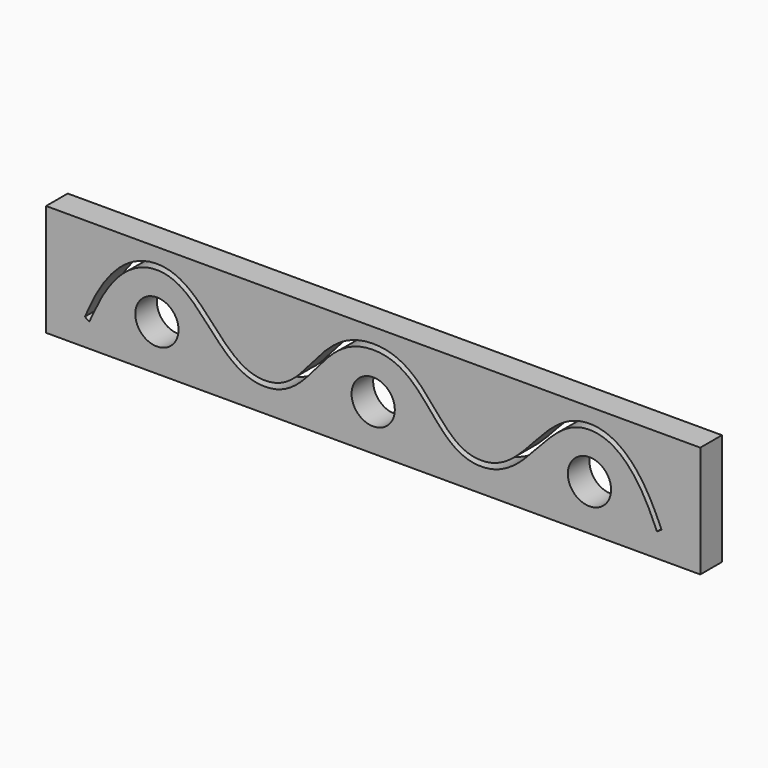
from build123d import *

# Parameters (mm, degrees)
F0_W     = 614.6593689919
F0_H     = 104.9060299742
F0_R     = 20.32
F1_DEPTH = 25.4


# Not quite as in the source:
# - ends of sketch curves that miss each other by under 0.0002 mm in the source are joined
# - the dataset's text gives a spline's control points without its knots; the knots are read off the source's solid


with BuildPart() as f1:
    # F0 (on Front) → F1 (new body)
    with BuildSketch(Plane.XZ):
        with Locations((0, 30.0749056167)):
            Rectangle(F0_W, F0_H)
        with Locations((-203.2, 20.4950086772)):
            Circle(F0_R, mode=Mode.SUBTRACT)
        with Locations((0, 20.4950086772)):
            Circle(F0_R, mode=Mode.SUBTRACT)
        with Locations((203.2, 20.4950086772)):
            Circle(F0_R, mode=Mode.SUBTRACT)
        with BuildLine():
            add(Edge.make_bspline(
                [(0, 63.5), (50.8, 63.5), (56.1175370932, 0), (101.6, 0)],
                knots=[0, 0, 0, 0, 119.8115603771, 119.8115603771, 119.8115603771, 119.8115603771], degree=3))
            add(Edge.make_bspline(
                [(0, 63.5), (-50.8, 63.5), (-56.1175370932, 0), (-101.6, 0)],
                knots=[0, 0, 0, 0, 119.8115603771, 119.8115603771, 119.8115603771, 119.8115603771], degree=3))
            add(Edge.make_bspline(
                [(-101.6, 0), (-147.0824629068, 0), (-161.2765789032, 63.5), (-203.2, 63.5)],
                knots=[0, 0, 0, 0, 119.8115603771, 119.8115603771, 119.8115603771, 119.8115603771], degree=3))
            add(Edge.make_bspline(
                [(-203.2, 63.5), (-244.3384826183, 63.5), (-263.5250381589, 4.789814353), (-266.7, 0)],
                knots=[0, 0, 0, 0, 89.8025612107, 89.8025612107, 89.8025612107, 89.8025612107], degree=3))
            Line((-266.7, 0), (-270.9370674539, 2.8072381066))
            add(Edge.make_bspline(
                [(-203.2, 68.58), (-206.0749247482, 68.58), (-211.6570572562, 68.0654677515), (-219.449703116, 65.9327946823), (-226.6139167838, 62.6573237184), (-235.3214664022, 57.0619610705), (-242.8084043286, 50.0452799381), (-249.2087272272, 42.3342188514), (-253.4945356129, 36.3678079721), (-257.2899146838, 30.3831174449), (-260.614540304, 24.5429222876), (-263.4845904473, 19.0110013278), (-265.5085267197, 14.7960229142), (-266.9118861506, 11.7464153334), (-267.8572021622, 9.6427688992), (-268.6955290239, 7.7460864416), (-269.4259857327, 6.0820696315), (-269.9424600992, 4.9140477877), (-270.2959565612, 4.1311962061), (-270.5287914392, 3.627286717), (-270.6926175205, 3.2849255658), (-270.8015436387, 3.065424442), (-270.8703935577, 2.930969375), (-270.9134306119, 2.8501874319), (-270.9322031409, 2.8160102358), (-270.9370674539, 2.8072381066)],
                knots=[0, 0, 0, 0, 0.062536818, 0.125073636, 0.1876104541, 0.2501472721, 0.3752209081, 0.4377577261, 0.5002945442, 0.5628313622, 0.6253681802, 0.6879049982, 0.7504418162, 0.7817102252, 0.8129786342, 0.8442470433, 0.8755154523, 0.9067838613, 0.9224180658, 0.9380522703, 0.9536864748, 0.961503577, 0.9693206793, 0.9771377815, 0.9803545729, 0.9803545729, 0.9803545729, 0.9803545729], degree=3))
            add(Edge.make_bspline(
                [(-101.6, 5.08), (-104.1471371, 5.08), (-108.9825494519, 5.5227985642), (-115.6526939013, 7.3372474831), (-121.9092103663, 10.1773367447), (-127.8642663749, 13.932751749), (-133.5886395499, 18.4728381682), (-140.9907545945, 25.3635161712), (-149.9577750737, 35.1135642507), (-159.0396450213, 45.1591389287), (-166.7656656648, 52.6297090899), (-172.9079254728, 57.7563865096), (-179.5208319726, 62.1967681684), (-186.7206430613, 65.7097554828), (-194.5808153214, 68.0207957165), (-200.2591817799, 68.58), (-203.2, 68.58)],
                knots=[0, 0, 0, 0, 0.0625, 0.125, 0.1875, 0.25, 0.3125, 0.375, 0.5, 0.625, 0.6875, 0.75, 0.8125, 0.875, 0.9375, 1, 1, 1, 1], degree=3))
            add(Edge.make_bspline(
                [(0, 68.58), (-3.4395833333, 68.58), (-9.9907230249, 68.0415568729), (-18.8754835158, 65.7852306257), (-26.8494717203, 62.2976627153), (-33.979773011, 57.8349170952), (-40.3831564519, 52.6526314317), (-48.14551851, 45.0924908704), (-56.7790114699, 34.9489891198), (-64.9188221861, 25.1689190997), (-71.5831601125, 18.303665252), (-76.7480703911, 13.8055020439), (-82.1704530142, 10.1054105506), (-87.9633960673, 7.3142638881), (-94.302168804, 5.5228017002), (-99.0528629, 5.08), (-101.6, 5.08)],
                knots=[0, 0, 0, 0, 0.0625, 0.125, 0.1875, 0.25, 0.3125, 0.375, 0.5, 0.625, 0.6875, 0.75, 0.8125, 0.875, 0.9375, 1, 1, 1, 1], degree=3))
            add(Edge.make_bspline(
                [(0, 68.58), (3.4395833333, 68.58), (9.9907230249, 68.0415568729), (18.8754835158, 65.7852306257), (26.8494717203, 62.2976627153), (33.979773011, 57.8349170952), (40.3831564519, 52.6526314317), (48.14551851, 45.0924908704), (56.7790114699, 34.9489891198), (64.9188221861, 25.1689190997), (71.5831601125, 18.303665252), (76.7480703911, 13.8055020439), (82.1704530142, 10.1054105506), (87.9633960673, 7.3142638881), (94.302168804, 5.5228017002), (99.0528629, 5.08), (101.6, 5.08)],
                knots=[0, 0, 0, 0, 0.0625, 0.125, 0.1875, 0.25, 0.3125, 0.375, 0.5, 0.625, 0.6875, 0.75, 0.8125, 0.875, 0.9375, 1, 1, 1, 1], degree=3))
            add(Edge.make_bspline(
                [(101.6, 5.08), (104.1471371, 5.08), (108.9825494519, 5.5227985642), (115.6526939013, 7.3372474831), (121.9092103663, 10.1773367447), (127.8642663749, 13.932751749), (133.5886395499, 18.4728381682), (140.9907545945, 25.3635161712), (149.9577750737, 35.1135642507), (159.0396450213, 45.1591389287), (166.7656656648, 52.6297090899), (172.9079254728, 57.7563865096), (179.5208319726, 62.1967681684), (186.7206430613, 65.7097554828), (194.5808153214, 68.0207957165), (200.2591817799, 68.58), (203.2, 68.58)],
                knots=[0, 0, 0, 0, 0.0625, 0.125, 0.1875, 0.25, 0.3125, 0.375, 0.5, 0.625, 0.6875, 0.75, 0.8125, 0.875, 0.9375, 1, 1, 1, 1], degree=3))
            add(Edge.make_bspline(
                [(203.2, 68.58), (206.0749247482, 68.58), (211.6570572562, 68.0654677515), (219.449703116, 65.9327946823), (226.6139167838, 62.6573237184), (235.3214664022, 57.0619610705), (242.8084043286, 50.0452799381), (249.2087272272, 42.3342188514), (253.4945356129, 36.3678079721), (257.2899146838, 30.3831174449), (260.614540304, 24.5429222876), (263.4845904473, 19.0110013278), (265.5085267197, 14.7960229142), (266.9118861506, 11.7464153334), (267.8572021622, 9.6427688992), (268.6955290239, 7.7460864416), (269.4259857327, 6.0820696315), (269.9424600992, 4.9140477877), (270.2959565612, 4.1311962061), (270.5287914392, 3.627286717), (270.6926175205, 3.2849255658), (270.8015436387, 3.065424442), (270.8703935577, 2.930969375), (270.9134306119, 2.8501874319), (270.9322031409, 2.8160102358), (270.9370672724, 2.8072380059)],
                knots=[0, 0, 0, 0, 0.062536818, 0.125073636, 0.1876104541, 0.2501472721, 0.3752209081, 0.4377577261, 0.5002945442, 0.5628313622, 0.6253681802, 0.6879049982, 0.7504418162, 0.7817102252, 0.8129786342, 0.8442470433, 0.8755154523, 0.9067838613, 0.9224180658, 0.9380522703, 0.9536864748, 0.961503577, 0.9693206793, 0.9771377815, 0.9803545729, 0.9803545729, 0.9803545729, 0.9803545729], degree=3))
            Line((270.9370672724, 2.8072380059), (266.7, 0))
            add(Edge.make_bspline(
                [(203.2, 63.5), (244.3384826183, 63.5), (263.5250381589, 4.789814353), (266.7, 0)],
                knots=[0, 0, 0, 0, 89.8025612107, 89.8025612107, 89.8025612107, 89.8025612107], degree=3))
            add(Edge.make_bspline(
                [(101.6, 0), (147.0824629068, 0), (161.2765789032, 63.5), (203.2, 63.5)],
                knots=[0, 0, 0, 0, 119.8115603771, 119.8115603771, 119.8115603771, 119.8115603771], degree=3))
        make_face(mode=Mode.SUBTRACT)
    extrude(amount=F1_DEPTH)


solid = f1.part
